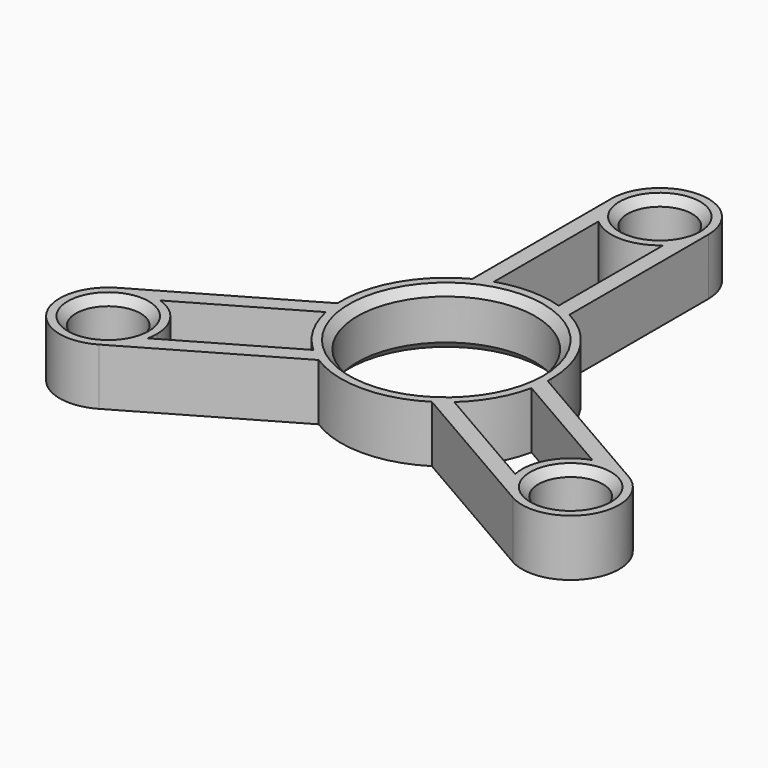
from build123d import *

# Parameters (mm, degrees)
F0_R     = 11
F0_R_2   = 4
F1_DEPTH = 3.5
F2_SIZE  = 1
F4_DEPTH = 7.001


# Not quite as in the source:
# - a feature names something its author has since deleted; it is built from what else it names


with BuildPart() as f1:
    # F0 (on Top) → F1 (new body, symmetric)
    with BuildSketch(Plane.XY):
        with BuildLine():
            ThreePointArc((-6, 11.5325625947), (0, 13), (6, 11.5325625947))
            Line((6, 11.5325625947), (6, 33))
            ThreePointArc((6, 33), (0, 27), (-6, 33))
            Line((-6, 33), (-6, 11.5325625947))
        make_face()
        with BuildLine():
            ThreePointArc((-6.9874921777, -10.96243372), (-11.2583302492, -6.5), (-12.9874921777, -0.5701288746))
            Line((-12.9874921777, -0.5701288746), (-31.5788383249, -11.3038475773))
            ThreePointArc((-31.5788383249, -11.3038475773), (-25.5788383249, -11.3038475773), (-22.5788383249, -16.5))
            ThreePointArc((-22.5788383249, -16.5), (-23.3826859022, -19.5), (-25.5788383249, -21.6961524227))
            Line((-25.5788383249, -21.6961524227), (-6.9874921777, -10.96243372))
        make_face()
        with BuildLine():
            Line((31.5788383249, -11.3038475773), (12.9874921777, -0.5701288746))
            ThreePointArc((12.9874921777, -0.5701288746), (11.2583302492, -6.5), (6.9874921777, -10.96243372))
            Line((6.9874921777, -10.96243372), (25.5788383249, -21.6961524227))
            ThreePointArc((25.5788383249, -21.6961524227), (23.3826859022, -13.5), (31.5788383249, -11.3038475773))
        make_face()
        with BuildLine():
            ThreePointArc((12.9874921777, -0.5701288746), (12.9968726683, -0.2851330301), (13, 0))
            ThreePointArc((13, 0), (11.1130553854, 6.7453687816), (6, 11.5325625947))
            ThreePointArc((6, 11.5325625947), (0, 13), (-6, 11.5325625947))
            ThreePointArc((-6, 11.5325625947), (-11.2583302492, 6.5), (-12.9874921777, -0.5701288746))
            ThreePointArc((-12.9874921777, -0.5701288746), (-11.2583302492, -6.5), (-6.9874921777, -10.96243372))
            ThreePointArc((-6.9874921777, -10.96243372), (0, -13), (6.9874921777, -10.96243372))
            ThreePointArc((6.9874921777, -10.96243372), (11.2583302492, -6.5), (12.9874921777, -0.5701288746))
        make_face()
        Circle(F0_R, mode=Mode.SUBTRACT)
        with BuildLine():
            ThreePointArc((-6, 33), (0, 27), (6, 33))
            ThreePointArc((6, 33), (0, 39), (-6, 33))
        make_face()
        with Locations((0, 33)):
            Circle(F0_R_2, mode=Mode.SUBTRACT)
        with BuildLine():
            ThreePointArc((-22.5788383249, -16.5), (-25.5788383249, -11.3038475773), (-31.5788383249, -11.3038475773))
            ThreePointArc((-31.5788383249, -11.3038475773), (-33.7749907476, -19.5), (-25.5788383249, -21.6961524227))
            ThreePointArc((-25.5788383249, -21.6961524227), (-23.3826859022, -19.5), (-22.5788383249, -16.5))
        make_face()
        with Locations((-28.5788383249, -16.5)):
            Circle(F0_R_2, mode=Mode.SUBTRACT)
        with BuildLine():
            ThreePointArc((34.5788383249, -16.5), (33.7749907476, -13.5), (31.5788383249, -11.3038475773))
            ThreePointArc((31.5788383249, -11.3038475773), (23.3826859022, -13.5), (25.5788383249, -21.6961524227))
            ThreePointArc((25.5788383249, -21.6961524227), (31.5788383249, -21.6961524227), (34.5788383249, -16.5))
        make_face()
        with Locations((28.5788383249, -16.5)):
            Circle(F0_R_2, mode=Mode.SUBTRACT)
    extrude(amount=F1_DEPTH, both=True)

    # F2
    f2_edges = [f1.edges().sort_by_distance(p)[0] for p in [
        (-4, 33, 3.5),
        (-11, 0, 3.5),
        (-32.578838, -16.5, 3.5),
        (24.578838, -16.5, 3.5),
        (-32.578838, -16.5, -3.5),
        (-11, 0, -3.5),
        (24.578838, -16.5, -3.5),
        (-4, 33, -3.5),
    ]]
    chamfer(f2_edges, length=F2_SIZE)

    # F3 (on face) → F4 (cut, through all)
    with BuildSketch(Plane.XY.offset(3.5)):
        with BuildLine():
            Line((4, 12.3693168769), (4, 28.527864045))
            ThreePointArc((4, 28.527864045), (0, 27), (-4, 28.527864045))
            Line((-4, 28.527864045), (-4, 12.3693168769))
            ThreePointArc((-4, 12.3693168769), (0, 13), (4, 12.3693168769))
        make_face()
        with BuildLine():
            ThreePointArc((-8.7121426428, -9.6487600536), (-11.2583302492, -6.5), (-12.7121426428, -2.7205568233))
            Line((-12.7121426428, -2.7205568233), (-26.7058549787, -10.7998304074))
            ThreePointArc((-26.7058549787, -10.7998304074), (-23.7189051938, -12.9813283811), (-22.5788383249, -16.5))
            ThreePointArc((-22.5788383249, -16.5), (-22.6106769632, -17.117292444), (-22.7058549787, -17.7280336376))
            Line((-22.7058549787, -17.7280336376), (-8.7121426428, -9.6487600536))
        make_face()
        with BuildLine():
            Line((26.7058549787, -10.7998304074), (12.7121426428, -2.7205568233))
            ThreePointArc((12.7121426428, -2.7205568233), (11.2583302492, -6.5), (8.7121426428, -9.6487600536))
            Line((8.7121426428, -9.6487600536), (22.7058549787, -17.7280336376))
            ThreePointArc((22.7058549787, -17.7280336376), (23.3826859022, -13.5), (26.7058549787, -10.7998304074))
        make_face()
    extrude(amount=-F4_DEPTH, mode=Mode.SUBTRACT)


solid = f1.part
